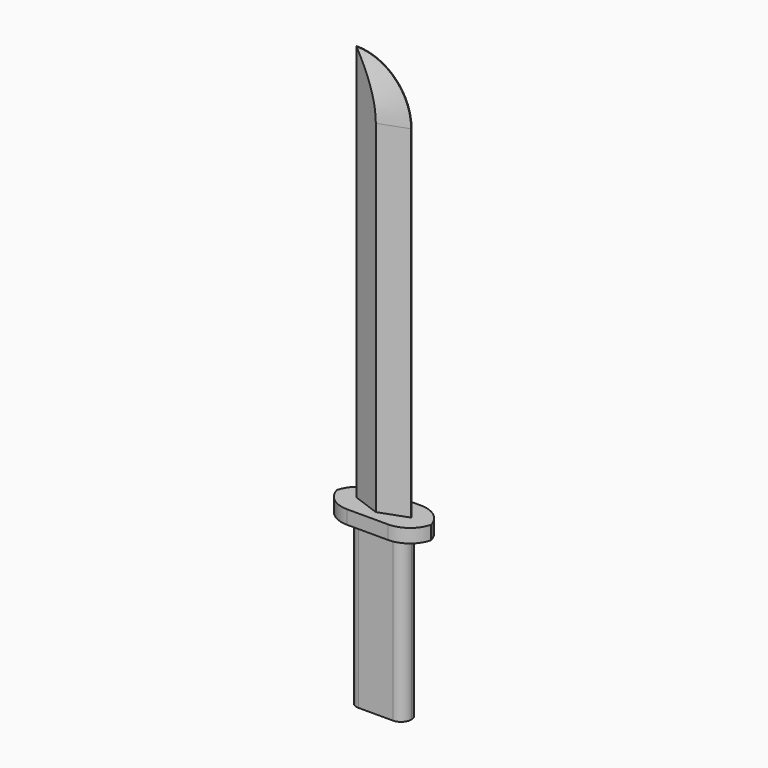
from build123d import *

# Parameters (mm, degrees)
F1_DEPTH     = 19.05
F2_W         = 88.9
F2_H         = 38.1
F3_DEPTH     = 12.7
F4_W         = 50.8
F4_H         = 381
F5_DEPTH     = 19.05
F6_R         = 50.79999
F7_T1_DEPTH  = 434.1925462068
F7_T3_DEPTH  = 317.50001
F7_T5_DEPTH  = 65.8925562068
F7_T8_ANGLE  = 90
F7_T10_ANGLE = 90
F8_R         = 9.52499
F9_T1_DEPTH  = 139.7


# Not quite as in the source:
# - a fillet or chamfer that OpenCascade refuses, or shapes differently, is made with other operations: its cross-section is extruded or revolved along the edge and cut away or added
# - a fillet or chamfer is up to 0.001 mm smaller than in the source, because OpenCascade refuses the exact size


with BuildPart() as f1:
    # F0 (on Front) → F1 (new body)
    with BuildSketch(Plane.XZ):
        Polygon((-25.4, -86.237093463), (0, -86.237093463), (25.4, -86.237093463), (25.4, 66.162906537), (-25.4, 66.162906537), align=None)
    extrude(amount=F1_DEPTH)

    # F2 (on face) → F3 (join)
    with BuildSketch(Plane.XY.offset(66.162906537)):
        with Locations((0, -9.525)):
            Rectangle(F2_W, F2_H)
    extrude(amount=F3_DEPTH)

    # F4 (on face) → F5 (join)
    with BuildSketch(Plane(origin=(0, 0, 0), x_dir=(-1, 0, 0), z_dir=(0, 1, 0))):
        with Locations((0, 256.662906537)):
            Rectangle(F4_W, F4_H)
    extrude(amount=-F5_DEPTH)

    # F6 (radius 50.8 in the source; OpenCascade refuses exactly that, so slightly less here)
    f6_edges = [f1.edges().sort_by_distance(p)[0] for p in [
        (25.4, -9.525, 447.162907),
    ]]
    fillet(f6_edges, radius=F6_R)

    # F7: chamfer of 25.4 x 9.2448439504 on 6 edges, made by hand

    # F7_s2 → F7_t1 (cut)
    with BuildSketch(Plane.XY.offset(78.862906537)):
        Polygon((0, 0), (-25.4, -9.2448439504), (-25.4, 0), align=None)
        Polygon((0, -19.05), (-25.4, -9.8051560496), (-25.4, -19.05), align=None)
    extrude(amount=F7_T1_DEPTH, mode=Mode.SUBTRACT)

    # F7_s4 → F7_t3 (cut)
    with BuildSketch(Plane.XY.offset(78.862906537)):
        Polygon((25.4, -9.2448439504), (0, 0), (25.4, 0), align=None)
        Polygon((25.4, -9.8051560496), (0, -19.05), (25.4, -19.05), align=None)
    extrude(amount=F7_T3_DEPTH, mode=Mode.SUBTRACT)

    # F7_s6 → F7_t5 (cut)
    with BuildSketch(Plane.YZ.offset(-91.2925462068)):
        Polygon((-19.05, 421.762906537), (-9.8051560496, 447.162906537), (-19.05, 447.162906537), align=None)
        Polygon((0, 421.762906537), (-9.2448439504, 447.162906537), (0, 447.162906537), align=None)
    extrude(amount=F7_T5_DEPTH, mode=Mode.SUBTRACT)

    # F7_s7 → F7_t8 (revolve, cut)
    with BuildSketch(Plane.XY.offset(396.362916537)):
        Polygon((0, 0), (25.4, -9.2448439504), (25.4, 0), align=None)
    revolve(axis=Axis((-25.39999, 0, 396.362916537), (0, -1, 0)), revolution_arc=F7_T8_ANGLE, mode=Mode.SUBTRACT)

    # F7_s9 → F7_t10 (revolve, cut)
    with BuildSketch(Plane.XY.offset(396.362916537)):
        Polygon((25.4, -9.8051560496), (0, -19.05), (25.4, -19.05), align=None)
    revolve(axis=Axis((-25.39999, -19.05, 396.362916537), (0, -1, 0)), revolution_arc=F7_T10_ANGLE, mode=Mode.SUBTRACT)

    # F8 (radius 9.525 in the source; OpenCascade refuses exactly that, so slightly less here)
    f8_edges = [f1.edges().sort_by_distance(p)[0] for p in [
        (25.4, 0, -10.037093),
        (-25.4, 0, -10.037093),
        (-25.4, -19.05, -10.037093),
        (25.4, -19.05, -10.037093),
    ]]
    fillet(f8_edges, radius=F8_R)

    # F9: fillet of radius 25.4 on 4 edges, made by hand

    # F9_s2 → F9_t1 (cut)
    with BuildSketch(Plane.XY.offset(2.662906537)):
        with BuildLine():
            ThreePointArc((19.05, -28.575), (37.0105122421, -21.1355122421), (44.45, -3.175))
            Line((44.45, -3.175), (44.45, -28.575))
            Line((44.45, -28.575), (19.05, -28.575))
        make_face()
        with BuildLine():
            ThreePointArc((19.05, 9.525), (37.0105122421, 2.0855122421), (44.45, -15.875))
            Line((44.45, -15.875), (44.45, 9.525))
            Line((44.45, 9.525), (19.05, 9.525))
        make_face()
        with BuildLine():
            ThreePointArc((-44.45, -3.175), (-37.0105122421, -21.1355122421), (-19.05, -28.575))
            Line((-19.05, -28.575), (-44.45, -28.575))
            Line((-44.45, -28.575), (-44.45, -3.175))
        make_face()
        with BuildLine():
            ThreePointArc((-44.45, -15.875), (-37.0105122421, 2.0855122421), (-19.05, 9.525))
            Line((-19.05, 9.525), (-44.45, 9.525))
            Line((-44.45, 9.525), (-44.45, -15.875))
        make_face()
    extrude(amount=F9_T1_DEPTH, mode=Mode.SUBTRACT)


solid = f1.part
